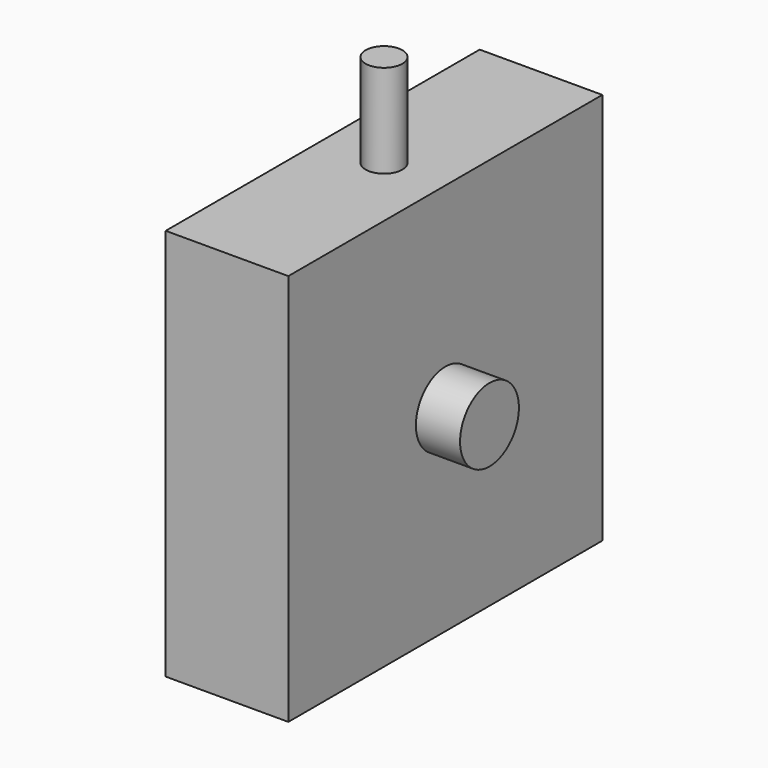
from build123d import *

# Parameters (mm, degrees)
F0_W     = 160
F0_H     = 160
F0_R     = 15
F1_DEPTH = 50
F2_T     = -10
F3_DEPTH = 65
F4_R     = 7.5
F5_DEPTH = 35
F6_DEPTH = 38
F7_R     = 7.5
F8_DEPTH = 68


with BuildPart() as f1:
    # F0 (on Right) → F1 (new body)
    with BuildSketch(Plane.YZ):
        with Locations((0, -80)):
            Rectangle(F0_W, F0_H)
        with Locations((0, -80)):
            Circle(F0_R, mode=Mode.SUBTRACT)
        with Locations((0, -80)):
            Circle(F0_R)
    extrude(amount=F1_DEPTH)

    # F2
    f2_openings = [f1.faces().sort_by_distance(p)[0] for p in [
        (25, 0, -160),
        (0, 0, -80),
    ]]
    offset(amount=F2_T, openings=f2_openings)

    # F0 (on Right) → F3 (cut)
    with BuildSketch(Plane.YZ):
        with Locations((0, -80)):
            Circle(F0_R)
    extrude(amount=F3_DEPTH, mode=Mode.SUBTRACT)

    # F4 (on face) → F5 (cut)
    with BuildSketch(Plane.XY):
        with Locations((25, 0)):
            Circle(F4_R)
    extrude(amount=-F5_DEPTH, mode=Mode.SUBTRACT)


with BuildPart() as f6:
    # F4 (on face) → F6 (new body, symmetric)
    with BuildSketch(Plane.XY):
        with Locations((25, 0)):
            Circle(F4_R)
    extrude(amount=F6_DEPTH, both=True)

    # F7
    f7_edges = [f6.edges().sort_by_distance(p)[0] for p in [
        (17.5, 0, -38),
    ]]
    fillet(f7_edges, radius=F7_R)


with BuildPart() as f8:
    # F0 (on Right) → F8 (new body)
    with BuildSketch(Plane.YZ):
        with Locations((0, -80)):
            Circle(F0_R)
    extrude(amount=F8_DEPTH)


solid = Compound([f1.part, f6.part, f8.part])
